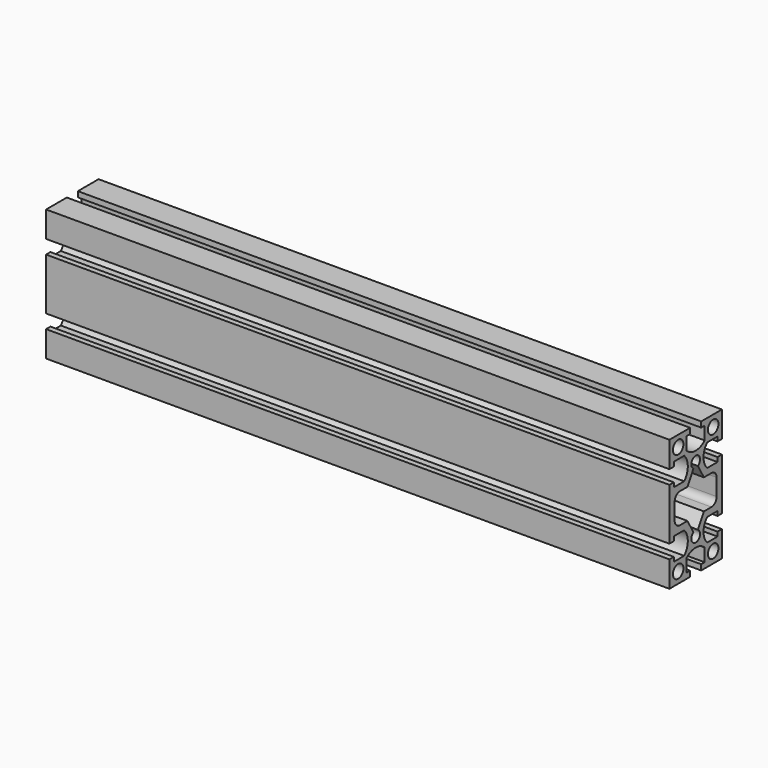
from build123d import *

# Parameters (mm, degrees)
F0_R     = 3
F1_DEPTH = 285


# Not quite as in the source:
# - ends of sketch curves that miss each other by under 0.0002 mm in the source are joined


with BuildPart() as f1:
    # F0 (on Right) → F1 (new body)
    with BuildSketch(Plane.YZ):
        with BuildLine():
            Line((12.5, -11.85), (15, -11.85))
            Line((15, -11.85), (15, 11.85))
            Line((15, 11.85), (12.5, 11.85))
            Line((12.5, 11.85), (12.5, 9.85))
            Line((12.5, 9.85), (6.547707, 9.85))
            ThreePointArc((6.5477069495, 9.8499999523), (4.5, 15), (6.5477069495, 20.1500000477))
            Line((6.547707, 20.15), (12.5, 20.15))
            Line((12.5, 20.15), (12.5, 18.15))
            Line((12.5, 18.15), (15, 18.15))
            Line((15, 18.15), (15, 30))
            Line((15, 30), (3.15, 30))
            Line((3.15, 30), (3.15, 27.5))
            Line((3.15, 27.5), (5.15, 27.5))
            Line((5.15, 27.5), (5.15, 21.547707))
            ThreePointArc((5.1500000477, 21.5477069495), (0, 19.5), (-5.1500000477, 21.5477069495))
            Line((-5.15, 21.547707), (-5.15, 27.5))
            Line((-5.15, 27.5), (-3.15, 27.5))
            Line((-3.15, 27.5), (-3.15, 30))
            Line((-3.15, 30), (-15, 30))
            Line((-15, 30), (-15, 18.15))
            Line((-15, 18.15), (-12.5, 18.15))
            Line((-12.5, 18.15), (-12.5, 20.15))
            Line((-12.5, 20.15), (-6.547707, 20.15))
            ThreePointArc((-6.5477069495, 20.1500000477), (-4.5, 15), (-6.5477069495, 9.8499999523))
            Line((-6.547707, 9.85), (-12.5, 9.85))
            Line((-12.5, 9.85), (-12.5, 11.85))
            Line((-12.5, 11.85), (-15, 11.85))
            Line((-15, 11.85), (-15, -11.85))
            Line((-15, -11.85), (-12.5, -11.85))
            Line((-12.5, -11.85), (-12.5, -9.85))
            Line((-12.5, -9.85), (-6.547707, -9.85))
            ThreePointArc((-6.5477069495, -9.8499999523), (-4.5, -15), (-6.5477069495, -20.1500000477))
            Line((-6.547707, -20.15), (-12.5, -20.15))
            Line((-12.5, -20.15), (-12.5, -18.15))
            Line((-12.5, -18.15), (-15, -18.15))
            Line((-15, -18.15), (-15, -30))
            Line((-15, -30), (-3.15, -30))
            Line((-3.15, -30), (-3.15, -27.5))
            Line((-3.15, -27.5), (-5.15, -27.5))
            Line((-5.15, -27.5), (-5.15, -21.547707))
            ThreePointArc((-5.1500000477, -21.5477069495), (0, -19.5), (5.1500000477, -21.5477069495))
            Line((5.15, -21.547707), (5.15, -27.5))
            Line((5.15, -27.5), (3.15, -27.5))
            Line((3.15, -27.5), (3.15, -30))
            Line((3.15, -30), (15, -30))
            Line((15, -30), (15, -18.15))
            Line((15, -18.15), (12.5, -18.15))
            Line((12.5, -18.15), (12.5, -20.15))
            Line((12.5, -20.15), (6.547707, -20.15))
            ThreePointArc((6.5477069495, -20.1500000477), (4.5, -15), (6.5477069495, -9.8499999523))
            Line((6.547707, -9.85), (12.5, -9.85))
            Line((12.5, -9.85), (12.5, -11.85))
        make_face()
        with Locations((-10, -25)):
            Circle(F0_R, mode=Mode.SUBTRACT)
        with Locations((10, -25)):
            Circle(F0_R, mode=Mode.SUBTRACT)
        with Locations((-10, 25)):
            Circle(F0_R, mode=Mode.SUBTRACT)
        with BuildLine():
            ThreePointArc((-12, 3.85), (-11.1213203436, 5.9713203436), (-9, 6.85))
            Line((-9, 6.85), (-4.705405, 6.85))
            Line((-4.705405, 6.85), (-1.25, 12.834936))
            ThreePointArc((-1.25, 12.834936), (0, 17.5), (1.2499997876, 12.8349363679))
            Line((1.2499997876, 12.8349363679), (4.705405, 6.85))
            Line((4.705405, 6.85), (9, 6.85))
            ThreePointArc((9, 6.85), (11.1213203436, 5.9713203436), (12, 3.85))
            Line((12, 3.85), (12, -3.85))
            ThreePointArc((12, -3.85), (11.1213203436, -5.9713203436), (9, -6.85))
            Line((9, -6.85), (4.705405, -6.85))
            Line((4.705405, -6.85), (1.25, -12.834937))
            ThreePointArc((1.25, -12.834937), (0, -17.5), (-1.2500002206, -12.8349366179))
            Line((-1.2500002206, -12.8349366179), (-4.705405, -6.85))
            Line((-4.705405, -6.85), (-9, -6.85))
            ThreePointArc((-9, -6.85), (-11.1213203436, -5.9713203436), (-12, -3.85))
            Line((-12, -3.85), (-12, 3.85))
        make_face(mode=Mode.SUBTRACT)
        with Locations((10, 25)):
            Circle(F0_R, mode=Mode.SUBTRACT)
    extrude(amount=F1_DEPTH)


solid = f1.part
